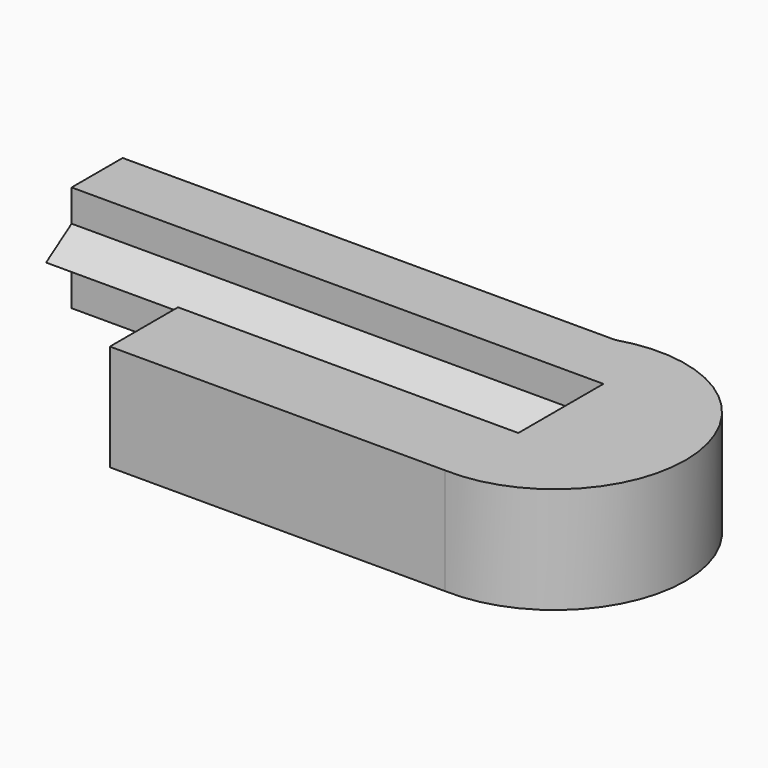
from build123d import *

# Parameters (mm, degrees)
F1_DEPTH = 1.27
F3_DEPTH = 12.7
F6_DEPTH = 1.778


with BuildPart() as f1:
    # F0 (on Top) → F1 (new body, symmetric)
    with BuildSketch(Plane.XY):
        with BuildLine():
            Line((0, 1.524), (0, 0))
            Line((0, 0), (12.7, 0))
            Line((12.7, 0), (12.7, -2.54))
            Line((12.7, -2.54), (4.572, -2.54))
            Line((4.572, -2.54), (4.572, -4.572))
            Line((4.572, -4.572), (12.5717104354, -4.572))
            ThreePointArc((12.5717104354, -4.572), (15.7940682602, -1.0438103752), (11.7644204026, 1.524))
            Line((11.7644204026, 1.524), (0, 1.524))
        make_face()
    extrude(amount=F1_DEPTH, both=True)

    # F2 (on face) → F3 (join, through all)
    with BuildSketch(Plane(origin=(0, 0, 0), x_dir=(0, -1, 0), z_dir=(-1, 0, 0))):
        Polygon((0.762, 0), (0, 0.508), (0, -0.508), align=None)
    extrude(amount=-F3_DEPTH)

    # F5 (on face) → F6 (join)
    with BuildSketch(Plane(origin=(3.81, 0, 0), x_dir=(0, -1, 0), z_dir=(-1, 0, 0))):
        Polygon((-4.064, -1.27), (-1.524, -1.27), (-1.524, 1.27), align=None)
    extrude(amount=-F6_DEPTH)


solid = f1.part
